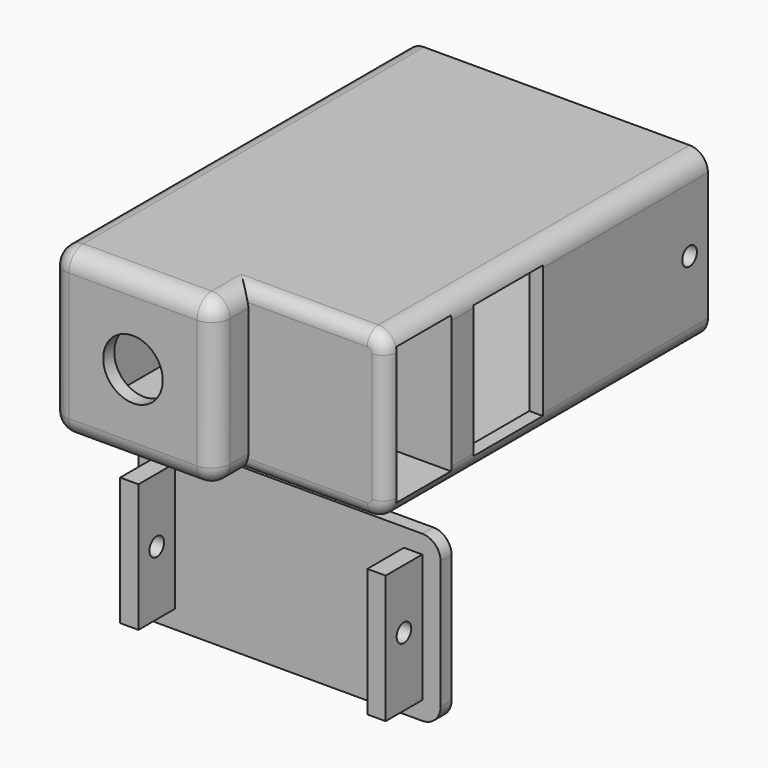
from build123d import *

# Parameters (mm, degrees)
F0_W          = 15
F0_H          = 15
F1_DEPTH      = 13.5
F0_R          = 6
F2_DEPTH      = 13.5
F0_R_2        = 4.5
F3_DEPTH      = 12
F5_DEPTH      = 15
F6_DEPTH      = 1.5
F7_DEPTH      = 35
F8_W          = 1.5
F8_H          = 15
F9_DEPTH      = 15
F10_W         = 2
F10_H         = 15
F11_DEPTH     = 15
F13_DEPTH     = 35
F14_W         = 1.5
F14_H         = 15
F15_DEPTH     = 33
F16_W         = 33
F16_H         = 18
F17_DEPTH     = 1.5
F16_W_2       = 2
F16_H_2       = 14
F18_DEPTH     = 6.5
F20_R         = 1
F21_DEPTH     = 1.5
F22_R         = 1
F23_DEPTH     = 1.5
F20_R_2       = 3.125
F24_DEPTH     = 1.5
F26_DEPTH     = 0.7
F27_R         = 1
F28_DEPTH     = 2
F29_DEPTH     = 5
F30_DEPTH     = 2
F32_DEPTH     = 13.5
F33_DEPTH     = 12
F0_R_3        = 3.25
F34_DEPTH     = 13.5
F35_DEPTH     = 12
F37_DEPTH     = 1.5
F38_T4_DEPTH  = 15
F38_T10_DEPTH = 15
F38_T16_DEPTH = 15
F38_T23_DEPTH = 15
F38_T29_DEPTH = 15
F38_T32_DEPTH = 2.5
F38_T34_DEPTH = 14
F38_T36_DEPTH = 14
F38_T38_DEPTH = 51.5
F38_T40_DEPTH = 54
F38_S44_W     = 2
F38_S44_H     = 2
F38_T45_DEPTH = 2
F38_S50_W     = 2
F38_S50_H     = 2
F38_T51_DEPTH = 2
F38_S56_W     = 2
F38_S56_H     = 2
F38_T57_DEPTH = 2
F38_S62_W     = 2
F38_S62_H     = 2
F38_T63_DEPTH = 2
F38_2_F1_R    = 2
F38_2_F2_R    = 2
F38_2_F3_R    = 2
F38_2_F4_R    = 2
F19_R         = 1
F40_DEPTH     = 2
F42_R         = 1.49999


# Not quite as in the source:
# - a fillet or chamfer that OpenCascade refuses, or shapes differently, is made with other operations: its cross-section is extruded or revolved along the edge and cut away or added
# - two fillets or chamfers of one size are made in one step
# - a fillet or chamfer is up to 0.001 mm smaller than in the source, because OpenCascade refuses the exact size
# - a feature names something its author has since deleted; it is built from what else it names


with BuildPart() as f1:
    # F0 (on Front) → F1 (new body)
    with BuildSketch(Plane.XZ):
        Polygon((16.5, 14.5), (16.5, 16), (-1.5, 16), (-1.5, -2), (16.5, -2), (16.5, -0.5), align=None)
        with Locations((7.5, 7)):
            Rectangle(F0_W, F0_H, mode=Mode.SUBTRACT)
    extrude(amount=F1_DEPTH)

    # F0 (on Front) → F2 (join)
    with BuildSketch(Plane.XZ):
        with Locations((7.5, 7)):
            Rectangle(F0_W, F0_H)
        with Locations((7.5, 7)):
            Circle(F0_R, mode=Mode.SUBTRACT)
    extrude(amount=F2_DEPTH)

    # F0 (on Front) → F3 (cut)
    with BuildSketch(Plane.XZ):
        with Locations((7.5, 7)):
            Rectangle(F0_W, F0_H)
        with Locations((7.5, 7)):
            Circle(F0_R, mode=Mode.SUBTRACT)
        with Locations((7.5, 7)):
            Circle(F0_R)
        with Locations((7.5, 7)):
            Circle(F0_R_2, mode=Mode.SUBTRACT)
    extrude(amount=F3_DEPTH, mode=Mode.SUBTRACT)

    # F4 (on face) → F5 (join)
    with BuildSketch(Plane.YZ.offset(16.5)):
        Polygon((0, -2), (0, -0.5), (-7.5, -0.5), (-7.5, 14.5), (0, 14.5), (0, 16), (-9, 16), (-9, -2), align=None)
    extrude(amount=F5_DEPTH)

    # F6 (cut): a face of the model
    f6_faces = [f1.faces().sort_by_distance(p)[0] for p in [
        (16.5, -3.75, 7),
    ]]
    extrude(f6_faces, amount=-F6_DEPTH, mode=Mode.SUBTRACT)

    # F0 (on Front) → F7 (join)
    with BuildSketch(Plane.XZ):
        Polygon((16.5, 14.5), (16.5, 16), (-1.5, 16), (-1.5, -2), (16.5, -2), (16.5, -0.5), align=None)
        with Locations((7.5, 7)):
            Rectangle(F0_W, F0_H, mode=Mode.SUBTRACT)
        Polygon((33, 16), (16.5, 16), (16.5, 14.5), (31.5, 14.5), (31.5, -0.5), (16.5, -0.5), (16.5, -2), (33, -2), align=None)
    extrude(amount=-F7_DEPTH)

    # F8 (on face) → F9 (cut)
    with BuildSketch(Plane(origin=(0, 35, 0), x_dir=(-1, 0, 0), z_dir=(0, 1, 0))):
        with Locations((-15.75, 7)):
            Rectangle(F8_W, F8_H)
    extrude(amount=-F9_DEPTH, mode=Mode.SUBTRACT)

    # F10 (on face) → F11 (join)
    with BuildSketch(Plane(origin=(31.5, 0, 0), x_dir=(0, -1, 0), z_dir=(-1, 0, 0))):
        with Locations((-1, 7)):
            Rectangle(F10_W, F10_H)
    extrude(amount=F11_DEPTH)

    # F12 (on face) → F13 (cut)
    with BuildSketch(Plane(origin=(0, 35, 0), x_dir=(-1, 0, 0), z_dir=(0, 1, 0))):
        Polygon((-31.5, -2), (-31.5, -0.5), (-31.5, 14.5), (-31.5, 16), (-33, 16), (-33, -2), align=None)
    extrude(amount=-F13_DEPTH, mode=Mode.SUBTRACT)

    # F14 (on face) → F15 (join)
    with BuildSketch(Plane(origin=(0, 2, 0), x_dir=(-1, 0, 0), z_dir=(0, 1, 0))):
        with Locations((-30.75, 7)):
            Rectangle(F14_W, F14_H)
    extrude(amount=F15_DEPTH)

    # F20 (on face) → F21 (cut)
    with BuildSketch(Plane(origin=(-1.5, 0, 0), x_dir=(0, -1, 0), z_dir=(-1, 0, 0))):
        with Locations((-32.5, 7)):
            Circle(F20_R)
    extrude(amount=-F21_DEPTH, mode=Mode.SUBTRACT)

    # F22 (on face) → F23 (cut)
    with BuildSketch(Plane.YZ.offset(31.5)):
        with Locations((32.5, 7)):
            Circle(F22_R)
    extrude(amount=-F23_DEPTH, mode=Mode.SUBTRACT)

    # F20 (on face) → F24 (cut)
    with BuildSketch(Plane(origin=(-1.5, 0, 0), x_dir=(0, -1, 0), z_dir=(-1, 0, 0))):
        with Locations((-24.875, 7)):
            Circle(F20_R_2)
    extrude(amount=-F24_DEPTH, mode=Mode.SUBTRACT)

    # F25 (on face) → F26 (cut)
    with BuildSketch(Plane(origin=(0, -12, 0), x_dir=(-1, 0, 0), z_dir=(0, 1, 0))):
        with BuildLine():
            Line((-14.4160797831, 6), (-13.4160797831, 6))
            ThreePointArc((-13.4160797831, 6), (-13.5, 7), (-13.4160797831, 8))
            Line((-13.4160797831, 8), (-14.4160797831, 8))
            Line((-14.4160797831, 8), (-14.4160797831, 7))
            Line((-14.4160797831, 7), (-14.4160797831, 6))
        make_face()
    extrude(amount=-F26_DEPTH, mode=Mode.SUBTRACT)

    # F29 (cut): a face of the model
    f29_faces = [f1.faces().sort_by_distance(p)[0] for p in [
        (15.75, 20, 7),
    ]]
    extrude(f29_faces, amount=-F29_DEPTH, mode=Mode.SUBTRACT)

    # F30 (cut): a face of the model
    f30_faces = [f1.faces().sort_by_distance(p)[0] for p in [
        (15, 7.5, 7),
    ]]
    extrude(f30_faces, amount=-F30_DEPTH, mode=Mode.SUBTRACT)

    # F31: union 

    # F0 (on Front) → F32 (join)
    with BuildSketch(Plane.XZ):
        with Locations((7.5, 7)):
            Circle(F0_R)
        with Locations((7.5, 7)):
            Circle(F0_R_2, mode=Mode.SUBTRACT)
    extrude(amount=F32_DEPTH)

    # F0 (on Front) → F33 (cut)
    with BuildSketch(Plane.XZ):
        with Locations((7.5, 7)):
            Circle(F0_R)
        with Locations((7.5, 7)):
            Circle(F0_R_2, mode=Mode.SUBTRACT)
    extrude(amount=F33_DEPTH, mode=Mode.SUBTRACT)

    # F0 (on Front) → F34 (join)
    with BuildSketch(Plane.XZ):
        with Locations((7.5, 7)):
            Circle(F0_R_2)
        with Locations((7.5, 7)):
            Circle(F0_R_3, mode=Mode.SUBTRACT)
    extrude(amount=F34_DEPTH)

    # F0 (on Front) → F35 (cut)
    with BuildSketch(Plane.XZ):
        with Locations((7.5, 7)):
            Circle(F0_R_2)
        with Locations((7.5, 7)):
            Circle(F0_R_3, mode=Mode.SUBTRACT)
    extrude(amount=F35_DEPTH, mode=Mode.SUBTRACT)

    # F36 (on face) → F37 (cut)
    with BuildSketch(Plane.YZ.offset(31.5)):
        Polygon((3, 14.25), (3, 7), (3, -0.25), (7.75, -0.25), (12.5, -0.25), (12.5, 7), (12.5, 14.25), (7.75, 14.25), align=None)
    extrude(amount=-F37_DEPTH, mode=Mode.SUBTRACT)

    # F38: fillet of radius 2 on 11 edges, made by hand


with BuildPart() as f17:
    # F16 (on Front) → F17 (new body)
    with BuildSketch(Plane.XZ):
        with Locations((15, -15.5205413848)):
            Rectangle(F16_W, F16_H)
        Polygon((29.5, -23.0205413848), (0.5, -23.0205413848), (0, -23.0205413848), (0, -8.0205413848), (0.5, -8.0205413848), (29.5, -8.0205413848), (30, -8.0205413848), (30, -23.0205413848), align=None, mode=Mode.SUBTRACT)
        Polygon((0.5, -22.5205413848), (0.5, -23.0205413848), (29.5, -23.0205413848), (29.5, -22.5205413848), (27.5, -22.5205413848), (27.5, -8.5205413848), (29.5, -8.5205413848), (29.5, -8.0205413848), (0.5, -8.0205413848), (0.5, -8.5205413848), (2.5, -8.5205413848), (2.5, -22.5205413848), align=None)
        Polygon((29.5, -22.5205413848), (29.5, -23.0205413848), (30, -23.0205413848), (30, -8.0205413848), (29.5, -8.0205413848), (29.5, -8.5205413848), align=None)
        Polygon((0, -23.0205413848), (0.5, -23.0205413848), (0.5, -22.5205413848), (0.5, -8.5205413848), (0.5, -8.0205413848), (0, -8.0205413848), align=None)
    extrude(amount=F17_DEPTH)

    # F16 (on Front) → F18 (join)
    with BuildSketch(Plane.XZ):
        with Locations((1.5, -15.5205413848)):
            Rectangle(F16_W_2, F16_H_2)
        with Locations((28.5, -15.5205413848)):
            Rectangle(F16_W_2, F16_H_2)
    extrude(amount=F18_DEPTH)

    # F27 (on face) → F28 (cut)
    with BuildSketch(Plane(origin=(0.5, 0, 0), x_dir=(0, -1, 0), z_dir=(-1, 0, 0))):
        with Locations((4, -15.5205413848)):
            Circle(F27_R)
    extrude(amount=-F28_DEPTH, mode=Mode.SUBTRACT)

    # F38#2: fillet of radius 2 on 4 edges, made by hand

    # F38_2_f1
    f38_2_f1_edges = [f17.edges().sort_by_distance(p)[0] for p in [
        (31.5, -0.75, -24.5205413848),
    ]]
    fillet(f38_2_f1_edges, radius=F38_2_F1_R)

    # F38_2_f2
    f38_2_f2_edges = [f17.edges().sort_by_distance(p)[0] for p in [
        (31.5, -0.75, -6.5205413848),
    ]]
    fillet(f38_2_f2_edges, radius=F38_2_F2_R)

    # F38_2_f3
    f38_2_f3_edges = [f17.edges().sort_by_distance(p)[0] for p in [
        (-1.5, -0.75, -24.5205413848),
    ]]
    fillet(f38_2_f3_edges, radius=F38_2_F3_R)

    # F38_2_f4
    f38_2_f4_edges = [f17.edges().sort_by_distance(p)[0] for p in [
        (-1.5, -0.75, -6.5205413848),
    ]]
    fillet(f38_2_f4_edges, radius=F38_2_F4_R)

    # F19 (on face) → F40 (cut)
    with BuildSketch(Plane.YZ.offset(29.5)):
        with Locations((-4, -15.0205413848)):
            Circle(F19_R)
    extrude(amount=-F40_DEPTH, mode=Mode.SUBTRACT)


with BuildPart() as f38_tool2:
    # F38_s3 → F38_t4 (new body)
    with BuildSketch(Plane.XY.offset(-0.5)):
        with BuildLine():
            ThreePointArc((30, 4), (29.4142135624, 2.5857864376), (28, 2))
            Line((28, 2), (30, 2))
            Line((30, 2), (30, 4))
        make_face()
    extrude(amount=F38_T4_DEPTH)

    split(bisect_by=Plane.XZ.offset(-3), keep=Keep.BOTTOM)

    split(bisect_by=Plane.XY.offset(-0.25), keep=Keep.BOTTOM)


with BuildPart() as f1_1:
    add(f1.part)

    # F38_t1: union F38_tool2
    add(f38_tool2.part)


with BuildPart() as f38_tool8:
    # F38_s9 → F38_t10 (new body)
    with BuildSketch(Plane.XY.offset(-0.5)):
        with BuildLine():
            ThreePointArc((30, 4), (29.4142135624, 2.5857864376), (28, 2))
            Line((28, 2), (30, 2))
            Line((30, 2), (30, 4))
        make_face()
    extrude(amount=F38_T10_DEPTH)

    split(bisect_by=Plane.XZ.offset(-3), keep=Keep.TOP)

    split(bisect_by=Plane.XY.offset(-0.25), keep=Keep.BOTTOM)


with BuildPart() as f1_2:
    add(f1_1.part)

    # F38_t7: union F38_tool8
    add(f38_tool8.part)


with BuildPart() as f38_tool14:
    # F38_s15 → F38_t16 (new body)
    with BuildSketch(Plane.XY.offset(-0.5)):
        with BuildLine():
            ThreePointArc((30, 4), (29.4142135624, 2.5857864376), (28, 2))
            Line((28, 2), (30, 2))
            Line((30, 2), (30, 4))
        make_face()
    extrude(amount=F38_T16_DEPTH)

    split(bisect_by=Plane.XZ.offset(-3), keep=Keep.TOP)

    split(bisect_by=Plane.XY.offset(-0.25), keep=Keep.TOP)

    split(bisect_by=Plane.XY.offset(14.25), keep=Keep.BOTTOM)


with BuildPart() as f1_3:
    add(f1_2.part)

    # F38_t13: union F38_tool14
    add(f38_tool14.part)


with BuildPart() as f38_tool21:
    # F38_s22 → F38_t23 (new body)
    with BuildSketch(Plane.XY.offset(-0.5)):
        with BuildLine():
            ThreePointArc((30, 4), (29.4142135624, 2.5857864376), (28, 2))
            Line((28, 2), (30, 2))
            Line((30, 2), (30, 4))
        make_face()
    extrude(amount=F38_T23_DEPTH)

    split(bisect_by=Plane.XZ.offset(-3), keep=Keep.BOTTOM)

    split(bisect_by=Plane.XY.offset(14.25), keep=Keep.TOP)


with BuildPart() as f1_4:
    add(f1_3.part)

    # F38_t20: union F38_tool21
    add(f38_tool21.part)


with BuildPart() as f38_tool27:
    # F38_s28 → F38_t29 (new body)
    with BuildSketch(Plane.XY.offset(-0.5)):
        with BuildLine():
            ThreePointArc((30, 4), (29.4142135624, 2.5857864376), (28, 2))
            Line((28, 2), (30, 2))
            Line((30, 2), (30, 4))
        make_face()
    extrude(amount=F38_T29_DEPTH)

    split(bisect_by=Plane.XZ.offset(-3), keep=Keep.TOP)

    split(bisect_by=Plane.XY.offset(14.25), keep=Keep.TOP)


with BuildPart() as f1_5:
    add(f1_4.part)

    # F38_t26: union F38_tool27
    add(f38_tool27.part)

    # F38_s33 → F38_t32 (cut)
    with BuildSketch(Plane.XZ.offset(9)):
        with BuildLine():
            ThreePointArc((16.5, 14), (15.9142135624, 15.4142135624), (14.5, 16))
            Line((14.5, 16), (16.5, 16))
            Line((16.5, 16), (16.5, 14))
        make_face()
        with BuildLine():
            ThreePointArc((16.5, 0), (15.9142135624, -1.4142135624), (14.5, -2))
            Line((14.5, -2), (16.5, -2))
            Line((16.5, -2), (16.5, 0))
        make_face()
    extrude(amount=F38_T32_DEPTH, mode=Mode.SUBTRACT)

    # F38_s35 → F38_t34 (cut)
    with BuildSketch(Plane.XY):
        with BuildLine():
            ThreePointArc((16.5, -11.5), (15.9142135624, -12.9142135624), (14.5, -13.5))
            Line((14.5, -13.5), (16.5, -13.5))
            Line((16.5, -13.5), (16.5, -11.5))
        make_face()
        with BuildLine():
            ThreePointArc((-1.5, -11.5), (-0.9142135624, -12.9142135624), (0.5, -13.5))
            Line((0.5, -13.5), (-1.5, -13.5))
            Line((-1.5, -13.5), (-1.5, -11.5))
        make_face()
    extrude(amount=F38_T34_DEPTH, mode=Mode.SUBTRACT)

    # F38_s37 → F38_t36 (cut)
    with BuildSketch(Plane.YZ.offset(0.5)):
        with BuildLine():
            ThreePointArc((-13.5, 14), (-12.9142135624, 15.4142135624), (-11.5, 16))
            Line((-11.5, 16), (-13.5, 16))
            Line((-13.5, 16), (-13.5, 14))
        make_face()
        with BuildLine():
            ThreePointArc((-11.5, -2), (-12.9142135624, -1.4142135624), (-13.5, 0))
            Line((-13.5, 0), (-13.5, -2))
            Line((-13.5, -2), (-11.5, -2))
        make_face()
    extrude(amount=F38_T36_DEPTH, mode=Mode.SUBTRACT)

    # F38_s39 → F38_t38 (cut)
    with BuildSketch(Plane.XZ.offset(-40)):
        with BuildLine():
            ThreePointArc((-1.5, 14), (-0.9142135624, 15.4142135624), (0.5, 16))
            Line((0.5, 16), (-1.5, 16))
            Line((-1.5, 16), (-1.5, 14))
        make_face()
        with BuildLine():
            ThreePointArc((-1.5, 0), (-0.9142135624, -1.4142135624), (0.5, -2))
            Line((0.5, -2), (-1.5, -2))
            Line((-1.5, -2), (-1.5, 0))
        make_face()
    extrude(amount=F38_T38_DEPTH, mode=Mode.SUBTRACT)

    # F38_s41 → F38_t40 (cut)
    with BuildSketch(Plane.XZ.offset(-40)):
        with BuildLine():
            ThreePointArc((31.5, 14), (30.9142135624, 15.4142135624), (29.5, 16))
            Line((29.5, 16), (31.5, 16))
            Line((31.5, 16), (31.5, 14))
        make_face()
        with BuildLine():
            ThreePointArc((31.5, 0), (30.9142135624, -1.4142135624), (29.5, -2))
            Line((29.5, -2), (31.5, -2))
            Line((31.5, -2), (31.5, 0))
        make_face()
    extrude(amount=F38_T40_DEPTH, mode=Mode.SUBTRACT)


with BuildPart() as f38_tool43:
    # F38_s44 → F38_t45 (new body)
    with BuildSketch(Plane.YZ.offset(14.5)):
        with Locations((-12.5, 15)):
            Rectangle(F38_S44_W, F38_S44_H)
    extrude(amount=F38_T45_DEPTH)

    # F38_s46 → F38_t47 (revolve, cut)
    with BuildSketch(Plane(origin=(14.5, -11.5, 14), x_dir=(0, 0.7071067812, -0.7071067812), z_dir=(0, -0.7071067812, -0.7071067812))):
        with BuildLine():
            ThreePointArc((0, -2), (2, 0), (0, 2))
            Line((0, 2), (0, -2))
        make_face()
    revolve(axis=Axis((14.5, -11.5, 14), (1, 0, 0)), mode=Mode.SUBTRACT)


with BuildPart() as f1_6:
    add(f1_5.part)

    # F38_t42: cut F38_tool43
    add(f38_tool43.part, mode=Mode.SUBTRACT)


with BuildPart() as f38_tool49:
    # F38_s50 → F38_t51 (new body)
    with BuildSketch(Plane.YZ.offset(14.5)):
        with Locations((-12.5, -1)):
            Rectangle(F38_S50_W, F38_S50_H)
    extrude(amount=F38_T51_DEPTH)

    # F38_s52 → F38_t53 (revolve, cut)
    with BuildSketch(Plane(origin=(14.5, -11.5, 0), x_dir=(0, 0.7071067812, 0.7071067812), z_dir=(0, 0.7071067812, -0.7071067812))):
        with BuildLine():
            ThreePointArc((0, -2), (2, 0), (0, 2))
            Line((0, 2), (0, -2))
        make_face()
    revolve(axis=Axis((14.5, -11.5, 0), (1, 0, 0)), mode=Mode.SUBTRACT)


with BuildPart() as f1_7:
    add(f1_6.part)

    # F38_t48: cut F38_tool49
    add(f38_tool49.part, mode=Mode.SUBTRACT)


with BuildPart() as f38_tool55:
    # F38_s56 → F38_t57 (new body)
    with BuildSketch(Plane.YZ.offset(0.5)):
        with Locations((-12.5, 15)):
            Rectangle(F38_S56_W, F38_S56_H)
    extrude(amount=-F38_T57_DEPTH)

    # F38_s58 → F38_t59 (revolve, cut)
    with BuildSketch(Plane(origin=(0.5, -11.5, 14), x_dir=(0, 0.7071067812, -0.7071067812), z_dir=(0, 0.7071067812, 0.7071067812))):
        with BuildLine():
            ThreePointArc((0, -2), (2, 0), (0, 2))
            Line((0, 2), (0, -2))
        make_face()
    revolve(axis=Axis((0.5, -11.5, 14), (-1, 0, 0)), mode=Mode.SUBTRACT)


with BuildPart() as f1_8:
    add(f1_7.part)

    # F38_t54: cut F38_tool55
    add(f38_tool55.part, mode=Mode.SUBTRACT)


with BuildPart() as f38_tool61:
    # F38_s62 → F38_t63 (new body)
    with BuildSketch(Plane.XY):
        with Locations((-0.5, -12.5)):
            Rectangle(F38_S62_W, F38_S62_H)
    extrude(amount=-F38_T63_DEPTH)

    # F38_s64 → F38_t65 (revolve, cut)
    with BuildSketch(Plane(origin=(0.5, -11.5, 0), x_dir=(0.7071067812, 0.7071067812, 0), z_dir=(-0.7071067812, 0.7071067812, 0))):
        with BuildLine():
            ThreePointArc((0, -2), (2, 0), (0, 2))
            Line((0, 2), (0, -2))
        make_face()
    revolve(axis=Axis((0.5, -11.5, 0), (0, 0, -1)), mode=Mode.SUBTRACT)


with BuildPart() as f1_9:
    add(f1_8.part)

    # F38_t60: cut F38_tool61
    add(f38_tool61.part, mode=Mode.SUBTRACT)

    # F42 (radius 1.5 in the source; OpenCascade refuses exactly that, so slightly less here)
    f42_edges = [f1_9.edges().sort_by_distance(p)[0] for p in [
        (30.914214, -9, 15.414214),
        (22, -9, 16),
        (22, -9, -2),
        (30.914214, -9, -1.414214),
        (31.5, -9, 7),
    ]]
    fillet(f42_edges, radius=F42_R)


solid = Compound([f17.part, f1_9.part])
